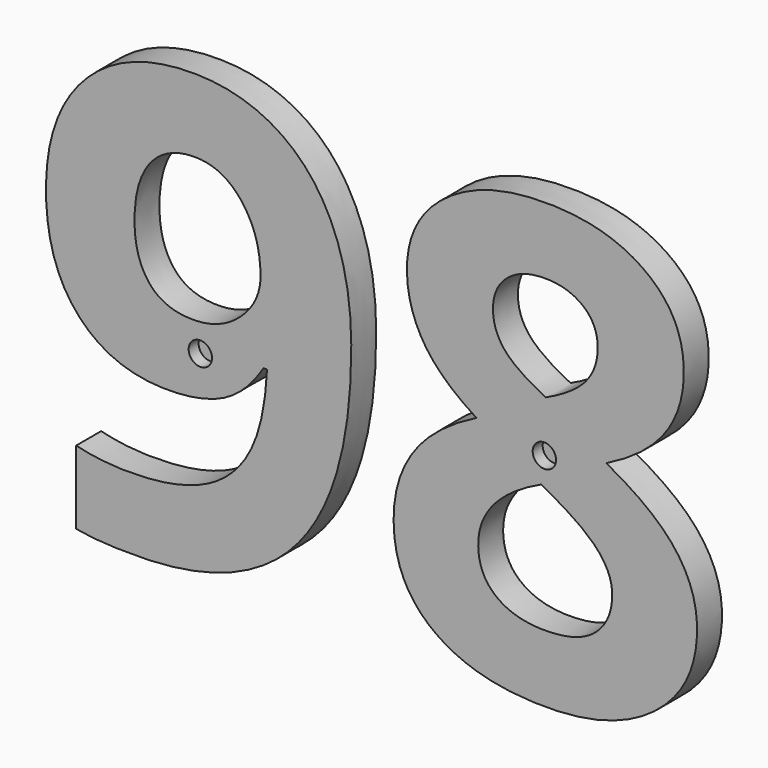
from build123d import *

# Parameters (mm, degrees)
F0_TEXT_SIZE = 123.4722222222
F1_DEPTH     = 6.35
F2_R         = 2.38125
F3_DEPTH     = 2.54


# Not quite as in the source:
# - a feature names something its author has since deleted; it is built from what else it names
# - Text() gives the source's letters only with a copy of the font that has no kerning and outlines rounded to 1/6400 em; it was checked with that copy


with BuildPart() as f1:
    # F0 (on Front) → F1 (new body)
    with BuildSketch(Plane.XZ):
        with Locations((0, 0)):
            Text('98', F0_TEXT_SIZE, font='Open Sans', font_style=FontStyle.BOLD, text_align=(TextAlign.LEFT, TextAlign.BOTTOM))
    extrude(amount=F1_DEPTH)

    # F2 (on face) → F3 (cut)
    with BuildSketch(Plane.XZ.offset(6.35)):
        with Locations((105.5428907275, 43.8017547131)):
            Circle(F2_R)
        with Locations((35.4241877794, 39.3011644483)):
            Circle(F2_R)
    extrude(amount=-F3_DEPTH, mode=Mode.SUBTRACT)


solid = f1.part
